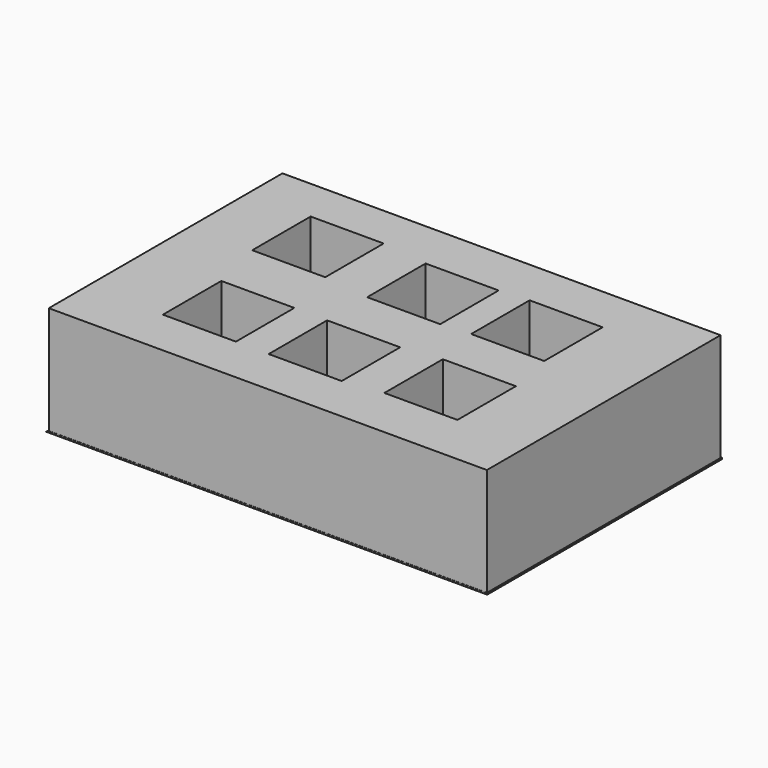
from build123d import *

# Parameters (mm, degrees)
F1_W         = 152.4
F1_H         = 101.6
F1_W_2       = 25.4
F1_H_2       = 25.4
F2_DEPTH     = 38.1
F3_W         = 153.4559056163
F3_H         = 102.0477414131
F3_W_2       = 152.4
F3_H_2       = 101.6
F4_DEPTH     = 0.508
F0_W         = 152.4
F0_H         = 101.6
F5_DEPTH     = 0.508
F6_T4_DEPTH  = 113.1193447297
F6_T9_DEPTH  = 113.1193447297
F6_T14_DEPTH = 113.1193447297


# Not quite as in the source:
# - a fillet or chamfer that OpenCascade refuses, or shapes differently, is made with other operations: its cross-section is extruded or revolved along the edge and cut away or added


with BuildPart() as f2:
    # F1 (on face) → F2 (new body)
    with BuildSketch(Plane.XY):
        Rectangle(F1_W, F1_H)
        with Locations((-36.918597445, -21.7081383014)):
            Rectangle(F1_W_2, F1_H_2, mode=Mode.SUBTRACT)
        with Locations((0, -21.855811876)):
            Rectangle(F1_W_2, F1_H_2, mode=Mode.SUBTRACT)
        with Locations((38.8383678732, -20.0837206056)):
            Rectangle(F1_W_2, F1_H_2, mode=Mode.SUBTRACT)
        with Locations((-41.6441853324, 23.0372088479)):
            Rectangle(F1_W_2, F1_H_2, mode=Mode.SUBTRACT)
        with Locations((0, 20.9697662408)):
            Rectangle(F1_W_2, F1_H_2, mode=Mode.SUBTRACT)
        with Locations((35.5895380648, 21.7081389993)):
            Rectangle(F1_W_2, F1_H_2, mode=Mode.SUBTRACT)
    extrude(amount=F2_DEPTH)

    # F3 (on face) → F4 (join)
    with BuildSketch(Plane.XY):
        with Locations((-0.3659911454, 0.1675821841)):
            Rectangle(F3_W, F3_H)
        Rectangle(F3_W_2, F3_H_2, mode=Mode.SUBTRACT)
    extrude(amount=F4_DEPTH)

    # F0 (on Top) → F5 (join)
    with BuildSketch(Plane.XY):
        Rectangle(F0_W, F0_H)
    extrude(amount=F5_DEPTH)

    # F6: fillet of radius 5.08 on 1 edges, made by hand


with BuildPart() as f6_tool2:
    # F6_s3 → F6_t4 (new body)
    with BuildSketch(Plane.XZ.offset(-56.7272545489)):
        with BuildLine():
            ThreePointArc((-74.8796232902, 0.508), (-76.0155458228, 0.3793715272), (-77.0939439535, 0))
            Line((-77.0939439535, 0), (-77.0939439535, 0.508))
            Line((-77.0939439535, 0.508), (-74.8796232902, 0.508))
        make_face()
    extrude(amount=F6_T4_DEPTH)

    split(bisect_by=Plane.XZ.offset(-50.8), keep=Keep.BOTTOM)


with BuildPart() as f2_1:
    add(f2.part)

    # F6_t1: cut F6_tool2
    add(f6_tool2.part, mode=Mode.SUBTRACT)


with BuildPart() as f6_tool7:
    # F6_s8 → F6_t9 (new body)
    with BuildSketch(Plane.XZ.offset(-56.7272545489)):
        with BuildLine():
            ThreePointArc((-74.8796232902, 0.508), (-76.0155458228, 0.3793715272), (-77.0939439535, 0))
            Line((-77.0939439535, 0), (-77.0939439535, 0.508))
            Line((-77.0939439535, 0.508), (-74.8796232902, 0.508))
        make_face()
    extrude(amount=F6_T9_DEPTH)

    split(bisect_by=Plane.YZ.offset(-76.2), keep=Keep.BOTTOM)


with BuildPart() as f2_2:
    add(f2_1.part)

    # F6_t6: cut F6_tool7
    add(f6_tool7.part, mode=Mode.SUBTRACT)


with BuildPart() as f6_tool12:
    # F6_s13 → F6_t14 (new body)
    with BuildSketch(Plane.XZ.offset(-56.7272545489)):
        with BuildLine():
            ThreePointArc((-74.8796232902, 0.508), (-76.0155458228, 0.3793715272), (-77.0939439535, 0))
            Line((-77.0939439535, 0), (-77.0939439535, 0.508))
            Line((-77.0939439535, 0.508), (-74.8796232902, 0.508))
        make_face()
    extrude(amount=F6_T14_DEPTH)

    split(bisect_by=Plane.XZ.offset(50.8), keep=Keep.TOP)


with BuildPart() as f2_3:
    add(f2_2.part)

    # F6_t11: cut F6_tool12
    add(f6_tool12.part, mode=Mode.SUBTRACT)


solid = f2_3.part
